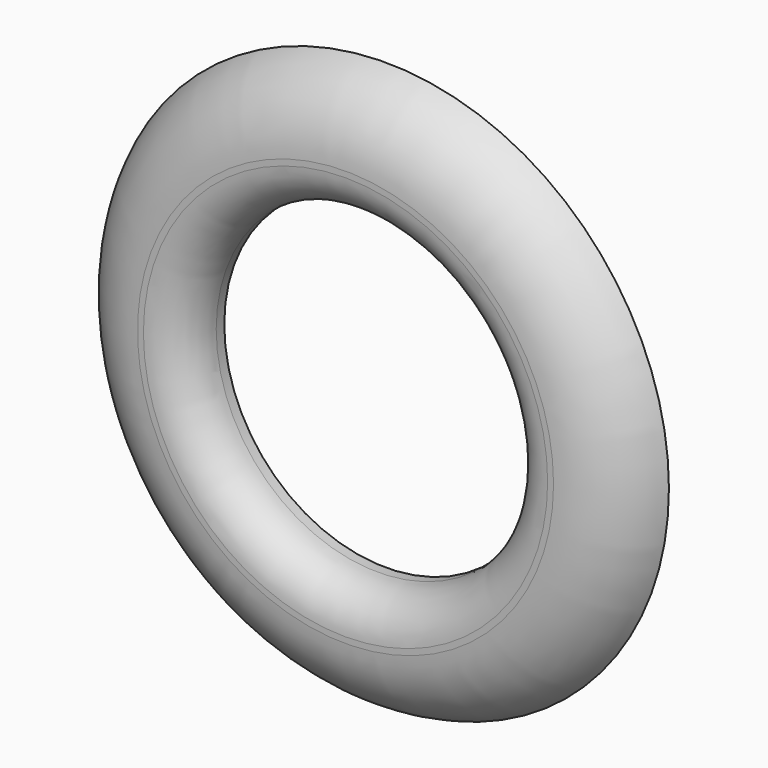
from build123d import *

# Parameters (mm, degrees)
F0_R     = 17.78
F0_R_2   = 10.16
F1_DEPTH = 3.175
F3_R     = 2.54


# Not quite as in the source:
# - a fillet or chamfer that OpenCascade refuses, or shapes differently, is made with other operations: its cross-section is extruded or revolved along the edge and cut away or added


with BuildPart() as f1:
    # F0 (on Front) → F1 (new body)
    with BuildSketch(Plane.XZ):
        Circle(F0_R)
        Circle(F0_R_2, mode=Mode.SUBTRACT)
    extrude(amount=F1_DEPTH)

    # F2: fillet of radius 5.08 on 1 edges, made by hand

    # F2_s1 → F2_t2 (revolve, cut)
    with BuildSketch(Plane.XY):
        with BuildLine():
            ThreePointArc((17.78, 0), (15.9105202921, -2.3071134838), (13.0707139607, -3.175))
            Line((13.0707139607, -3.175), (17.78, -3.175))
            Line((17.78, -3.175), (17.78, 0))
        make_face()
    revolve(axis=Axis((0, -3.175, 0), (0, -1, 0)), mode=Mode.SUBTRACT)

    # F3
    f3_edges = [f1.edges().sort_by_distance(p)[0] for p in [
        (-10.16, -3.175, 0),
    ]]
    fillet(f3_edges, radius=F3_R)


solid = f1.part
